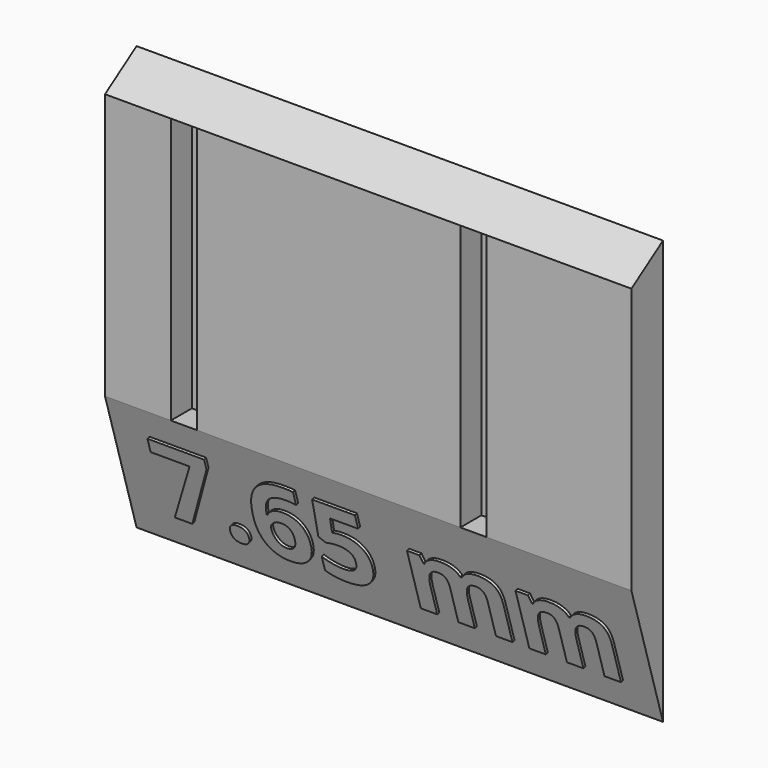
from build123d import *

# Parameters (mm, degrees)
F0_W         = 50.8
F0_H         = 25.654
F1_DEPTH     = 3.81
F2_W         = 2.54
F2_H         = 25.654
F3_DEPTH     = 2.54
F5_DEPTH     = 50.8
F6_TEXT_SIZE = 10.6695069311
F7_DEPTH     = 0.254


# Not quite as in the source:
# - Text() gives the source's letters only with a copy of the font that has no kerning and outlines rounded to 1/6400 em; it was checked with that copy


with BuildPart() as f1:
    # F0 (on Front) → F1 (new body)
    with BuildSketch(Plane.XZ):
        with Locations((9.5210788604, -2.5933608413)):
            Rectangle(F0_W, F0_H)
    extrude(amount=F1_DEPTH)

    # F2 (on face) → F3 (cut)
    with BuildSketch(Plane.XZ.offset(3.81)):
        with Locations((-8.2589211396, -2.5933608413)):
            Rectangle(F2_W, F2_H)
        with Locations((19.6810788604, -2.5933608413)):
            Rectangle(F2_W, F2_H)
    extrude(amount=-F3_DEPTH, mode=Mode.SUBTRACT)

    # F4 (on face) → F5 (join)
    with BuildSketch(Plane(origin=(-15.8789211396, 0, 0), x_dir=(0, -1, 0), z_dir=(-1, 0, 0))):
        Polygon((3.81, -15.4203608413), (0, -15.4203608413), (0, -28.1203608413), align=None)
        Polygon((0, 12.7736391587), (0, 10.2336391587), (3.81, 10.2336391587), align=None)
    extrude(amount=-F5_DEPTH)

    # F6 (on face) → F7 (join)
    with BuildSketch(Plane(origin=(0, -7.7395488554, -2.3218646566), x_dir=(1, 0, 0), z_dir=(0, -0.9578262852, -0.2873478856))):
        with Locations((-12.4897044152, -23.9504761994)):
            Text('7.65 mm', F6_TEXT_SIZE, font='Open Sans', font_style=FontStyle.BOLD, text_align=(TextAlign.LEFT, TextAlign.BOTTOM))
    extrude(amount=F7_DEPTH)


solid = f1.part
